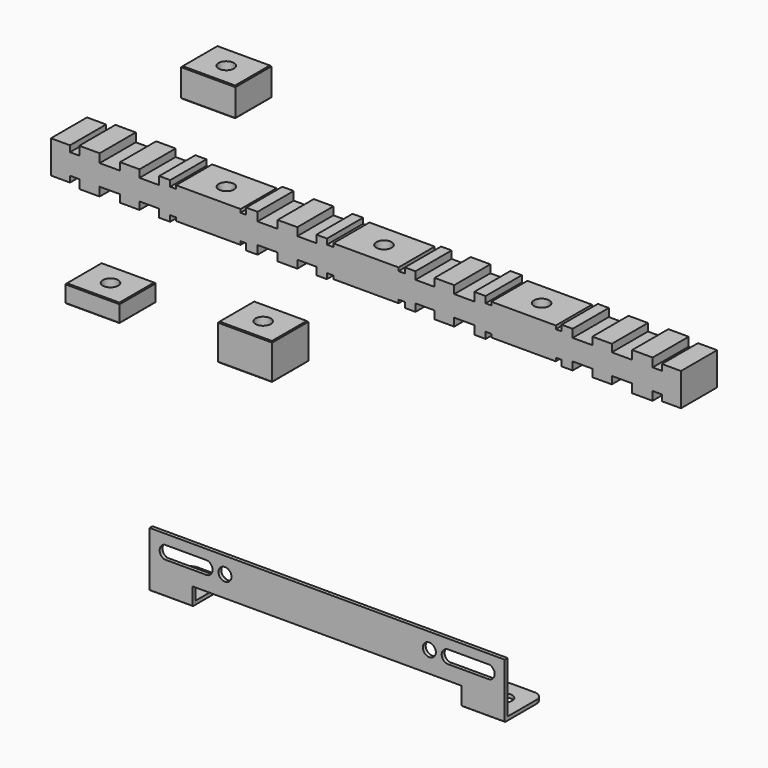
from build123d import *

# Parameters (mm, degrees)
F1_DEPTH  = 25
F2_W      = 30
F2_H      = 20
F3_DEPTH  = 25
F4_W      = 30
F4_H      = 16
F5_DEPTH  = 25
F6_W      = 30
F6_H      = 10
F7_DEPTH  = 25
F8_SIZE   = 0.5
F8_2_SIZE = 0.5
F8_3_SIZE = 0.5
F9_R      = 3.6028705458
F10_DEPTH = 2
F11_W     = 23.7871110439
F11_H     = 2
F11_W_2   = 23.7632221616
F11_H_2   = 1.9790753297
F12_DEPTH = 25
F13_R     = 0.5
F14_R     = 5
F15_R     = 4.25
F16_R     = 4.25
F17_DEPTH = 2.001
F20_R     = 4.25
F21_DEPTH = 76.3909049693
F19_R     = 4.25
F18_R     = 4.25
F22_DEPTH = 217.8817511064
F23_R     = 4.25
F24_DEPTH = 276.8010267333
F25_R     = 4.25
F27_DEPTH = 20
F26_R     = 4.25
F28_DEPTH = 25


with BuildPart() as f1:
    # F0 (on Front) → F1 (new body)
    with BuildSketch(Plane.XZ):
        Polygon((-156.9127636468, 14.8200338624), (-156.9127636468, 5.7359881692), (-156.9127636468, -3.348057524), (-146.3469222056, -3.348057524), (-146.3469222056, 0), (-141.2151361071, 0), (-141.2151361071, -4.8163233229), (-129.9238098947, -4.8163233229), (-129.9238098947, 0), (-118.632474036, 0), (-118.632474036, -4.1673955208), (-107.8602869303, -4.1673955208), (-107.8602869303, 0), (-96.9583078131, 0), (-96.9583078131, -4.4269659785), (-90.8583919597, -4.4269659785), (-90.8583919597, -1.1823308868), (-87.6137653086, -1.1823308868), (-87.6137653086, -2.999326502), (-51.9227708593, -2.999326502), (-51.9227708593, -1.1823308868), (-48.7857109655, -1.1823308868), (-48.7857109655, -4.7250164395), (-42.4892260512, -4.7250164395), (-42.4892260512, 0), (-31.3931135836, 0), (-31.3931135836, -4.3729061708), (-20.5111024682, -4.3729061708), (-20.5111024682, 0), (-9.9440986386, 0), (-9.9440986386, -4.1673955208), (-4.0986614626, -4.1673955208), (-4.0986614626, -1.1823308868), (-0.5792415786, -1.1823308868), (-0.5792415786, -2.999326502), (17.479924475, -2.999326502), (35.5390905287, -2.999326502), (35.5390905287, -1.1823308868), (39.0585104127, -1.1823308868), (39.0585104127, -4.1673955208), (44.9039475886, -4.1673955208), (44.9039475886, 0), (55.4709514183, 0), (55.4709514183, -4.3729061708), (66.3529625337, -4.3729061708), (66.3529625337, 0), (77.4490750013, 0), (77.4490750013, -4.7250164395), (83.7455599156, -4.7250164395), (83.7455599156, -1.1823308868), (86.8826198094, -1.1823308868), (86.8826198094, -2.999326502), (122.5736142587, -2.999326502), (122.5736142587, -1.1823308868), (125.8182409098, -1.1823308868), (125.8182409098, -4.4269659785), (131.9181567632, -4.4269659785), (131.9181567632, 0), (142.8201358804, 0), (142.8201358804, -4.1673955208), (153.5923229861, -4.1673955208), (153.5923229861, 0), (164.8836588448, 0), (164.8836588448, -4.8163233229), (176.1749850572, -4.8163233229), (176.1749850572, 0), (181.3067711557, 0), (181.3067711557, -3.348057524), (191.8726125969, -3.348057524), (191.8726125969, 5.7359881692), (191.8726125969, 14.8200338624), (181.3067711557, 14.8200338624), (181.3067711557, 11.4719763384), (176.1749850572, 11.4719763384), (176.1749850572, 16.2882996613), (164.8836588448, 16.2882996613), (164.8836588448, 11.4719763384), (153.5923229861, 11.4719763384), (153.5923229861, 15.6393718592), (142.8201358804, 15.6393718592), (142.8201358804, 11.4719763384), (131.9181567632, 11.4719763384), (131.9181567632, 15.8989423169), (125.8182409098, 15.8989423169), (125.8182409098, 12.6543072252), (122.5736142587, 12.6543072252), (122.5736142587, 14.4713028404), (86.8826198094, 14.4713028404), (86.8826198094, 12.6543072252), (83.7455599156, 12.6543072252), (83.7455599156, 16.1969927779), (77.4490750013, 16.1969927779), (77.4490750013, 11.4719763384), (66.3529625337, 11.4719763384), (66.3529625337, 15.8448825092), (55.4709514183, 15.8448825092), (55.4709514183, 11.4719763384), (44.9039475886, 11.4719763384), (44.9039475886, 15.6393718592), (39.0585104127, 15.6393718592), (39.0585104127, 12.6543072252), (35.5390905287, 12.6543072252), (35.5390905287, 14.4713028404), (17.479924475, 14.4713028404), (-0.5792415786, 14.4713028404), (-0.5792415786, 12.6543072252), (-4.0986614626, 12.6543072252), (-4.0986614626, 15.6393718592), (-9.9440986386, 15.6393718592), (-9.9440986386, 11.4719763384), (-20.5111024682, 11.4719763384), (-20.5111024682, 15.8448825092), (-31.3931135836, 15.8448825092), (-31.3931135836, 11.4719763384), (-42.4892260512, 11.4719763384), (-42.4892260512, 16.1969927779), (-48.7857109655, 16.1969927779), (-48.7857109655, 12.6543072252), (-51.9227708593, 12.6543072252), (-51.9227708593, 14.4713028404), (-87.6137653086, 14.4713028404), (-87.6137653086, 12.6543072252), (-90.8583919597, 12.6543072252), (-90.8583919597, 15.8989423169), (-96.9583078131, 15.8989423169), (-96.9583078131, 11.4719763384), (-107.8602869303, 11.4719763384), (-107.8602869303, 15.6393718592), (-118.632474036, 15.6393718592), (-118.632474036, 11.4719763384), (-129.9238098947, 11.4719763384), (-129.9238098947, 16.2882996613), (-141.2151361071, 16.2882996613), (-141.2151361071, 11.4719763384), (-146.3469222056, 11.4719763384), (-146.3469222056, 14.8200338624), align=None)
    extrude(amount=F1_DEPTH)

    # F20 (on face) → F21 (cut, through all)
    with BuildSketch(Plane(origin=(0, 0, -2.999326502), x_dir=(1, 0, 0), z_dir=(0, 0, -1))):
        with Locations((-69.7682680839, 12.5)):
            Circle(F20_R)
    extrude(amount=-F21_DEPTH, mode=Mode.SUBTRACT)

    # F19 (on face) + F18 (on face) → F22 (cut, through all)
    with BuildSketch(Plane.XY.offset(14.4713028404)):
        with Locations((17.479924475, -12.5)):
            Circle(F19_R)
    with BuildSketch(Plane.XY.offset(14.4713028404)):
        with Locations((104.728117034, -12.5)):
            Circle(F18_R)
    extrude(amount=-F22_DEPTH, mode=Mode.SUBTRACT)


with BuildPart() as f3:
    # F2 (on Front) → F3 (new body)
    with BuildSketch(Plane.XZ):
        with Locations((-49.4428929892, -54.479341954)):
            Rectangle(F2_W, F2_H)
    extrude(amount=F3_DEPTH)

    # F8
    f8_edges = [f3.edges().sort_by_distance(p)[0] for p in [
        (-49.442893, -25, -44.479342),
        (-34.442893, -12.5, -44.479342),
        (-64.442893, -12.5, -44.479342),
        (-49.442893, 0, -44.479342),
        (-64.442893, -12.5, -64.479342),
        (-34.442893, -12.5, -64.479342),
        (-49.442893, 0, -64.479342),
        (-49.442893, -25, -64.479342),
    ]]
    chamfer(f8_edges, length=F8_SIZE)

    # F25 (on face) → F27 (cut, through all)
    with BuildSketch(Plane(origin=(0, 0, -64.479341954), x_dir=(1, 0, 0), z_dir=(0, 0, -1))):
        with Locations((-49.4428929892, 12.5)):
            Circle(F25_R)
    extrude(amount=-F27_DEPTH, mode=Mode.SUBTRACT)


with BuildPart() as f5:
    # F4 (on Front) → F5 (new body)
    with BuildSketch(Plane.XZ):
        with Locations((-69.8153842241, 65.3905784673)):
            Rectangle(F4_W, F4_H)
    extrude(amount=F5_DEPTH)

    # F8#3
    f8_3_edges = [f5.edges().sort_by_distance(p)[0] for p in [
        (-54.815384, -12.5, 73.390578),
        (-84.815384, -12.5, 73.390578),
        (-69.815384, 0, 73.390578),
        (-69.815384, -25, 73.390578),
        (-84.815384, -12.5, 57.390578),
        (-54.815384, -12.5, 57.390578),
        (-69.815384, 0, 57.390578),
        (-69.815384, -25, 57.390578),
    ]]
    chamfer(f8_3_edges, length=F8_3_SIZE)

    # F23 (on face) → F24 (cut, through all)
    with BuildSketch(Plane.XY.offset(73.3905784673)):
        with Locations((-69.8153842241, -12.5)):
            Circle(F23_R)
    extrude(amount=-F24_DEPTH, mode=Mode.SUBTRACT)


with BuildPart() as f7:
    # F6 (on Front) → F7 (new body)
    with BuildSketch(Plane.XZ):
        with Locations((-133.9033134282, -58.2528847276)):
            Rectangle(F6_W, F6_H)
    extrude(amount=F7_DEPTH)

    # F8#2
    f8_2_edges = [f7.edges().sort_by_distance(p)[0] for p in [
        (-118.903313, -12.5, -53.252885),
        (-148.903313, -12.5, -53.252885),
        (-133.903313, 0, -53.252885),
        (-133.903313, -25, -53.252885),
        (-148.903313, -12.5, -63.252885),
        (-118.903313, -12.5, -63.252885),
        (-133.903313, 0, -63.252885),
        (-133.903313, -25, -63.252885),
    ]]
    chamfer(f8_2_edges, length=F8_2_SIZE)

    # F26 (on face) → F28 (cut)
    with BuildSketch(Plane(origin=(0, 0, -63.2528847276), x_dir=(1, 0, 0), z_dir=(0, 0, -1))):
        with Locations((-133.9033134282, 12.5)):
            Circle(F26_R)
    extrude(amount=-F28_DEPTH, mode=Mode.SUBTRACT)


with BuildPart() as f10:
    # F9 (on Front) → F10 (new body)
    with BuildSketch(Plane.XZ):
        Polygon((-22.3887339234, -172.7569699287), (-120.6744611263, -172.6086586714), (-120.6744611263, -203.1636536121), (-96.8873500824, -203.1636536121), (-96.8873500824, -193.3814436197), (-22.3887339234, -193.3814436197), align=None)
        with BuildLine():
            ThreePointArc((-89.4251316786, -178.1000308653), (-85.8103992128, -182.0202274237), (-90.0103312333, -185.3057719568))
            Line((-90.0103312333, -185.3057719568), (-112.2996848099, -185.3057719568))
            ThreePointArc((-112.2996848099, -185.3057719568), (-115.1180225225, -181.7029014111), (-112.2996848099, -178.1000308653))
            Line((-112.2996848099, -178.1000308653), (-89.4251316786, -178.1000308653))
        make_face(mode=Mode.SUBTRACT)
        with Locations((-78.9490147419, -181.7029014111)):
            Circle(F9_R, mode=Mode.SUBTRACT)
        Polygon((75.8969932795, -172.9052811861), (-22.3887339234, -172.7569699287), (-22.3887339234, -193.3814436197), (52.1098822355, -193.3814436197), (52.1098822355, -203.409448266), (75.8969932795, -203.409448266), align=None)
        with Locations((34.171546895, -181.7029014111)):
            Circle(F9_R, mode=Mode.SUBTRACT)
        with BuildLine():
            Line((67.522216963, -185.3057719568), (45.2328633864, -185.3057719568))
            ThreePointArc((45.2328633864, -185.3057719568), (41.0329313659, -182.0202274237), (44.6476638317, -178.1000308653))
            Line((44.6476638317, -178.1000308653), (67.522216963, -178.1000308653))
            ThreePointArc((67.522216963, -178.1000308653), (70.3405546756, -181.7029014111), (67.522216963, -185.3057719568))
        make_face(mode=Mode.SUBTRACT)
    extrude(amount=F10_DEPTH)

    # F11 (on face) → F12 (join)
    with BuildSketch(Plane(origin=(0, 0, 0), x_dir=(-1, 0, 0), z_dir=(0, 1, 0))):
        with Locations((-64.0034377575, -202.409448266)):
            Rectangle(F11_W, F11_H)
        with Locations((108.7928500456, -202.1741159473)):
            Rectangle(F11_W_2, F11_H_2)
    extrude(amount=F12_DEPTH)

    # F13
    f13_edges = [f10.edges().sort_by_distance(p)[0] for p in [
        (64.003438, 0, -201.409448),
        (-108.79285, 0, -201.184578),
        (64.003438, -2, -203.409448),
        (-108.780906, -2, -203.163654),
    ]]
    fillet(f13_edges, radius=F13_R)

    # F14
    f14_edges = [f10.edges().sort_by_distance(p)[0] for p in [
        (75.896993, 25, -202.409448),
        (52.109882, 25, -202.409448),
        (-96.911239, 25, -202.174116),
        (-120.674461, 25, -202.174116),
    ]]
    fillet(f14_edges, radius=F14_R)

    # F15 (on face) + F16 (on face) → F17 (cut, through all)
    with BuildSketch(Plane.XY.offset(-201.409448266)):
        with Locations((64.0034377575, 12.75)):
            Circle(F15_R)
    with BuildSketch(Plane.XY.offset(-201.1845782825)):
        with Locations((-108.7928500456, 12.75)):
            Circle(F16_R)
    extrude(amount=-F17_DEPTH, mode=Mode.SUBTRACT)


solid = Compound([f1.part, f3.part, f5.part, f7.part, f10.part])
